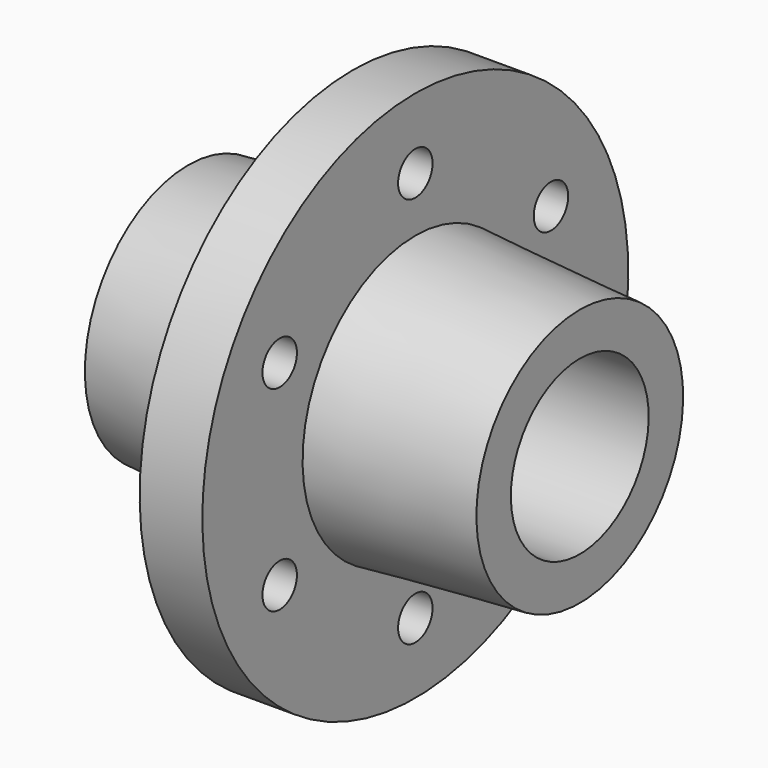
from build123d import *

# Parameters (mm, degrees)
F3_D            = 5.5
F3_COPIES_COUNT = 6


# Not quite as in the source:
# - a pattern or mirror of a feature is missing from the dataset's text; its kind, count and spacing are read off the source's solid


with BuildPart() as f1:
    # F0 (on Front) → F1 (revolve)
    with BuildSketch(Plane.XZ):
        Polygon((-25, 16.5), (-25, 11), (25, 11), (25, 16.5), (4, 18), (4, 34), (-4, 34), (-4, 18), align=None)
    revolve(axis=Axis((-2.8921069455, 0, 0), (1, 0, 0)))

    # F3 (through all)
    with Locations(Plane.YZ.offset(4)):
        with Locations((0, 25)):
            f3 = Hole(F3_D / 2)

    # F3_copies: F3 ×6 about axis
    f3_copies_axis = Axis((0, 0, 0), (1, 0, 0))
    for i in range(1, F3_COPIES_COUNT):
        add(f3.rotate(f3_copies_axis, i * 360 / F3_COPIES_COUNT), mode=Mode.SUBTRACT)


solid = f1.part
